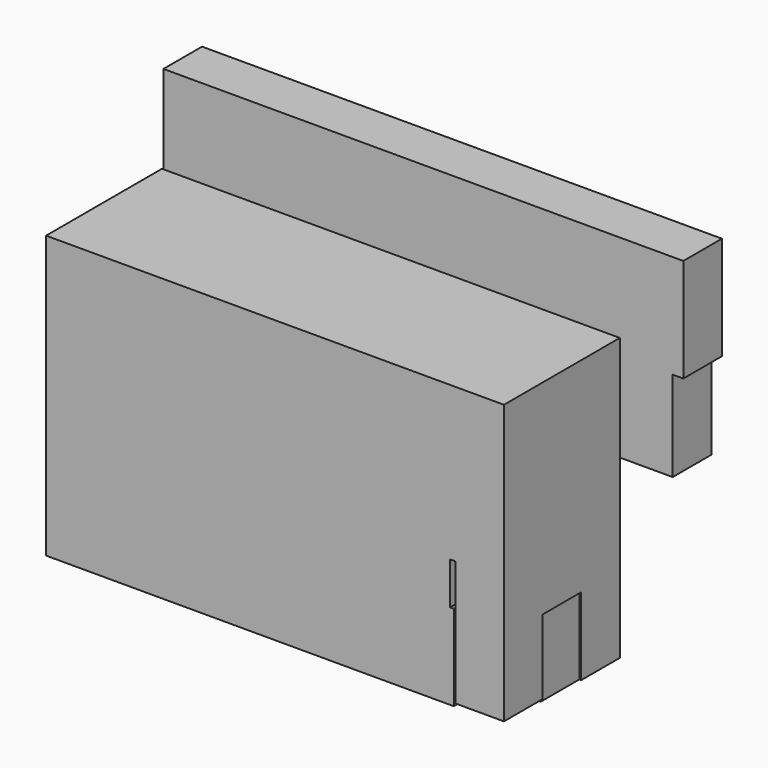
from build123d import *

# Parameters (mm, degrees)
F0_W      = 212.6203179359
F0_H      = 22.2269091755
F1_DEPTH  = 25.4
F2_W      = 13.6859714985
F2_H      = 40.4146937653
F3_DEPTH  = 25.4
F5_DEPTH  = 25.4
F7_DEPTH  = 25.4
F8_W      = 86.2983710408
F8_H      = 107.4658855796
F9_DEPTH  = 25.4
F10_W     = 85.29484272
F10_H     = 40.7659783959
F11_DEPTH = 25.4
F12_W     = 86.2983710408
F12_H     = 148.2318639755
F13_DEPTH = 25.4
F15_W     = 73.2594318688
F15_H     = 64.30112198
F15_H_2   = 9.4412900507
F15_W_2   = 48.5810935497
F15_H_3   = 47.4680401385
F15_W_3   = 54.1693717241
F15_H_4   = 43.5468889773
F16_DEPTH = 25.4


with BuildPart() as f1:
    # F0 (on Front) → F1 (new body)
    with BuildSketch(Plane.XZ):
        Polygon((-136.7080956697, 70.86391747), (-136.7080956697, -9.9654700607), (75.9122222662, -9.9654700607), (78.8259357214, -9.9654700607), (78.8259357214, 70.86391747), align=None)
        with Locations((-30.3979367018, -21.0789246485)):
            Rectangle(F0_W, F0_H)
        Polygon((75.9122222662, -32.1923792362), (-136.7080956697, -32.1923792362), (-136.7080956697, -77.3679465055), (77.8233259916, -77.3679465055), (77.8233259916, -32.1923792362), align=None)
    extrude(amount=F1_DEPTH)

    # F2 (on face) → F3 (join)
    with BuildSketch(Plane.YZ.offset(78.8259357214)):
        Polygon((0, 30.4492237046), (0, 70.86391747), (-25.4, 70.86391747), (-25.4, -75.8049190044), (0, -75.8049190044), (0, -9.9654700607), (-13.6859714985, -9.9654700607), (-13.6859714985, 30.4492237046), align=None)
        with Locations((-6.8429857492, 10.241876822)):
            Rectangle(F2_W, F2_H)
    extrude(amount=F3_DEPTH)

    # F4 (on face) → F5 (join)
    with BuildSketch(Plane(origin=(0, 0, 0), x_dir=(-1, 0, 0), z_dir=(0, 1, 0))):
        Polygon((75.8066177368, -40.0540344417), (75.8066177368, -77.3679465055), (136.7080956697, -77.3679465055), (136.7080956697, 70.86391747), (75.8066177368, 70.86391747), (75.8066177368, 35.8203239739), (99.0835726261, 35.8203239739), (99.0835726261, -40.0540344417), align=None)
        Polygon((-17.9275646806, -77.3679465055), (75.8066177368, -77.3679465055), (75.8066177368, -40.0540344417), (24.7398540378, -40.0540344417), (24.7398540378, 35.8203239739), (75.8066177368, 35.8203239739), (75.8066177368, 70.86391747), (-17.9275646806, 70.86391747), align=None)
    extrude(amount=F5_DEPTH)

    # F6 (on face) → F7 (join)
    with BuildSketch(Plane(origin=(0, 25.4, 0), x_dir=(-1, 0, 0), z_dir=(0, 1, 0))):
        Polygon((24.7398540378, -40.0540344417), (24.7398540378, 14.7684887052), (-17.9275646806, 14.7684887052), (-17.9275646806, -77.3679465055), (77.9451653361, -77.3679465055), (77.9451653361, -40.0540344417), align=None)
        Polygon((-17.9275646806, 14.7684887052), (24.7398540378, 14.7684887052), (24.7398540378, 35.8203239739), (77.9451653361, 35.8203239739), (77.9451653361, 70.86391747), (-17.9275646806, 70.86391747), align=None)
        Polygon((77.9451653361, 70.86391747), (77.9451653361, 35.8203239739), (99.0835726261, 35.8203239739), (99.0835726261, -40.0540344417), (77.9451653361, -40.0540344417), (77.9451653361, -77.3679465055), (136.7080956697, -77.3679465055), (136.7080956697, 70.86391747), align=None)
    extrude(amount=F7_DEPTH)

    # F8 (on face) → F9 (join)
    with BuildSketch(Plane(origin=(0, 0, 0), x_dir=(-1, 0, 0), z_dir=(0, 1, 0))):
        with Locations((-61.076750201, 17.1309746802)):
            Rectangle(F8_W, F8_H)
    extrude(amount=F9_DEPTH)

    # F10 (on face) → F11 (join)
    with BuildSketch(Plane(origin=(0, 0, 0), x_dir=(-1, 0, 0), z_dir=(0, 1, 0))):
        with Locations((-60.5749860406, -56.9849573076)):
            Rectangle(F10_W, F10_H)
    extrude(amount=F11_DEPTH)

    # F12 (on face) → F13 (join)
    with BuildSketch(Plane(origin=(0, 25.4, 0), x_dir=(-1, 0, 0), z_dir=(0, 1, 0))):
        with Locations((-61.076750201, -3.2520145178)):
            Rectangle(F12_W, F12_H)
    extrude(amount=F13_DEPTH)

    # F15 (on face) → F16 (join)
    with BuildSketch(Plane(origin=(0, 50.8, 0), x_dir=(-1, 0, 0), z_dir=(0, 1, 0))):
        Polygon((25.0786952674, -29.877435416), (25.0786952674, 34.423686564), (98.3381271362, 34.423686564), (98.3381271362, -29.877435416), (135.9246820211, -29.877435416), (135.9246820211, 117.3784919083), (-83.4680050611, 117.3784919083), (-83.4680050611, 73.831602931), (-83.4680050611, 62.8992691636), (-83.4680050611, 15.4312290251), (-83.4680050611, -29.877435416), align=None)
        with Locations((61.7084112018, 2.273125574)):
            Rectangle(F15_W, F15_H)
        with Locations((61.7084112018, -34.5980804414)):
            Rectangle(F15_W, F15_H_2)
        with Locations((-107.758551836, 39.1652490944)):
            Rectangle(F15_W_2, F15_H_3)
        Polygon((-132.0490986109, 62.8992691636), (-83.4680050611, 62.8992691636), (-83.4680050611, 73.831602931), (-137.6373767853, 73.831602931), (-137.6373767853, 62.8992691636), align=None)
        with Locations((-110.5526909232, 95.6050474197)):
            Rectangle(F15_W_3, F15_H_4)
    extrude(amount=F16_DEPTH)


solid = f1.part
